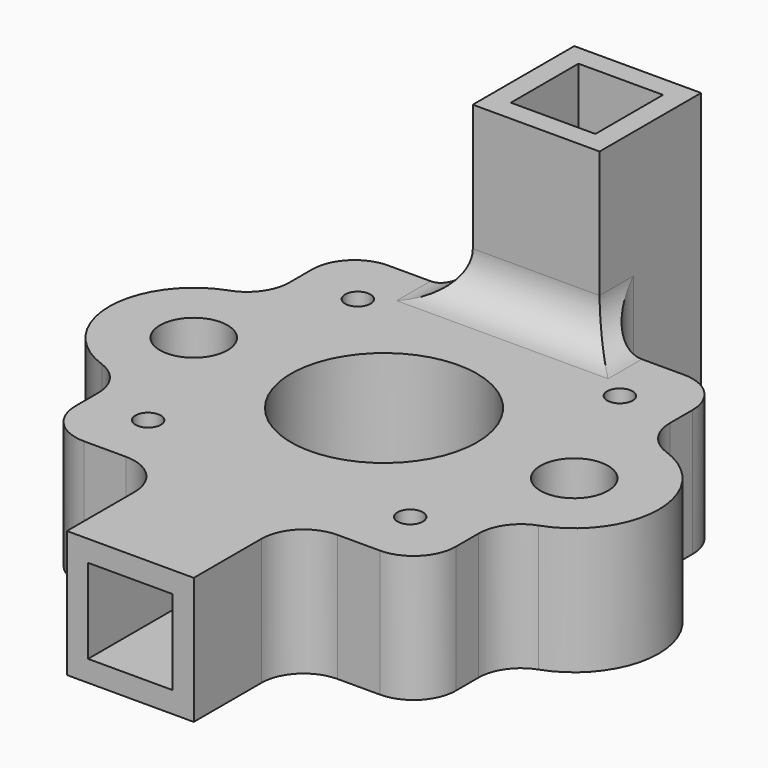
from build123d import *

# Parameters (mm, degrees)
F0_R     = 1.5
F0_R_2   = 11
F1_DEPTH = 15
F2_W     = 10
F2_H     = 10
F3_DEPTH = 20
F4_W     = 15
F4_H     = 15
F4_W_2   = 10
F4_H_2   = 10
F5_DEPTH = 20
F6_F1_R  = 5
F6_F2_R  = 5
F6_F3_R  = 5
F6_F4_R  = 5
F6_F5_R  = 5
F6_F6_R  = 5
F6_F7_R  = 5
F6_F8_R  = 5
F6_F9_R  = 5
F6_F10_R = 5
F6_F11_R = 5
F6_F12_R = 5
F6_F13_R = 5
F7_R     = 4
F8_DEPTH = 7.5
F9_R     = 5


with BuildPart() as f1:
    # F0 (on Top) → F1 (new body)
    with BuildSketch(Plane.XY):
        with BuildLine():
            Line((-45, -32.5), (-45, -45))
            Line((-45, -45), (-30, -45))
            Line((-30, -45), (-30, -60))
            Line((-30, -60), (-15, -60))
            Line((-15, -60), (-15, -45))
            Line((-15, -45), (0, -45))
            Line((0, -45), (0, -32.5))
            ThreePointArc((0, -32.5), (10, -22.5), (0, -12.5))
            Line((0, -12.5), (0, 0))
            Line((0, 0), (-15, 0))
            Line((-15, 0), (-15, 15))
            Line((-15, 15), (-30, 15))
            Line((-30, 15), (-30, 0))
            Line((-30, 0), (-45, 0))
            Line((-45, 0), (-45, -12.5))
            ThreePointArc((-45, -12.5), (-55, -22.5), (-45, -32.5))
        make_face()
        with Locations((-38, -38)):
            Circle(F0_R, mode=Mode.SUBTRACT)
        with Locations((-7, -38)):
            Circle(F0_R, mode=Mode.SUBTRACT)
        with Locations((-38, -7)):
            Circle(F0_R, mode=Mode.SUBTRACT)
        with Locations((-22.5, -22.5)):
            Circle(F0_R_2, mode=Mode.SUBTRACT)
        with Locations((-7, -7)):
            Circle(F0_R, mode=Mode.SUBTRACT)
    extrude(amount=F1_DEPTH)

    # F2 (on face) → F3 (cut)
    with BuildSketch(Plane.XZ.offset(60)):
        with Locations((-22.5, 7.5)):
            Rectangle(F2_W, F2_H)
    extrude(amount=-F3_DEPTH, mode=Mode.SUBTRACT)

    # F4 (on face) → F5 (join)
    with BuildSketch(Plane.XY.offset(15)):
        with Locations((-22.5, 7.5)):
            Rectangle(F4_W, F4_H)
        with Locations((-22.5, 7.5)):
            Rectangle(F4_W_2, F4_H_2, mode=Mode.SUBTRACT)
    extrude(amount=F5_DEPTH)

    # F6: fillet of radius 5 on 13 edges, made by hand

    # F6_f1
    f6_f1_edges = [f1.edges().sort_by_distance(p)[0] for p in [
        (-15, 0, 7.5),
    ]]
    fillet(f6_f1_edges, radius=F6_F1_R)

    # F6_f2
    f6_f2_edges = [f1.edges().sort_by_distance(p)[0] for p in [
        (-22.5, 0, 15),
    ]]
    fillet(f6_f2_edges, radius=F6_F2_R)

    # F6_f3
    f6_f3_edges = [f1.edges().sort_by_distance(p)[0] for p in [
        (0, -12.5, 7.5),
    ]]
    fillet(f6_f3_edges, radius=F6_F3_R)

    # F6_f4
    f6_f4_edges = [f1.edges().sort_by_distance(p)[0] for p in [
        (0, 0, 7.5),
    ]]
    fillet(f6_f4_edges, radius=F6_F4_R)

    # F6_f5
    f6_f5_edges = [f1.edges().sort_by_distance(p)[0] for p in [
        (0, -32.5, 7.5),
    ]]
    fillet(f6_f5_edges, radius=F6_F5_R)

    # F6_f6
    f6_f6_edges = [f1.edges().sort_by_distance(p)[0] for p in [
        (0, -45, 7.5),
    ]]
    fillet(f6_f6_edges, radius=F6_F6_R)

    # F6_f7
    f6_f7_edges = [f1.edges().sort_by_distance(p)[0] for p in [
        (-15, -45, 7.5),
    ]]
    fillet(f6_f7_edges, radius=F6_F7_R)

    # F6_f8
    f6_f8_edges = [f1.edges().sort_by_distance(p)[0] for p in [
        (-30, -45, 7.5),
    ]]
    fillet(f6_f8_edges, radius=F6_F8_R)

    # F6_f9
    f6_f9_edges = [f1.edges().sort_by_distance(p)[0] for p in [
        (-45, -45, 7.5),
    ]]
    fillet(f6_f9_edges, radius=F6_F9_R)

    # F6_f10
    f6_f10_edges = [f1.edges().sort_by_distance(p)[0] for p in [
        (-45, -32.5, 7.5),
    ]]
    fillet(f6_f10_edges, radius=F6_F10_R)

    # F6_f11
    f6_f11_edges = [f1.edges().sort_by_distance(p)[0] for p in [
        (-45, -12.5, 7.5),
    ]]
    fillet(f6_f11_edges, radius=F6_F11_R)

    # F6_f12
    f6_f12_edges = [f1.edges().sort_by_distance(p)[0] for p in [
        (-45, 0, 7.5),
    ]]
    fillet(f6_f12_edges, radius=F6_F12_R)

    # F6_f13
    f6_f13_edges = [f1.edges().sort_by_distance(p)[0] for p in [
        (-30, 0, 7.5),
    ]]
    fillet(f6_f13_edges, radius=F6_F13_R)

    # F7 (on face) → F8 (cut)
    with BuildSketch(Plane.XY.offset(15)):
        with Locations((-45, -22.5)):
            Circle(F7_R)
        with Locations((0, -22.5)):
            Circle(F7_R)
    extrude(amount=-F8_DEPTH, mode=Mode.SUBTRACT)

    # F9
    f9_edges = [f1.edges().sort_by_distance(p)[0] for p in [
        (-15, 0, 15),
        (-30, 0, 15),
    ]]
    fillet(f9_edges, radius=F9_R)


solid = f1.part
